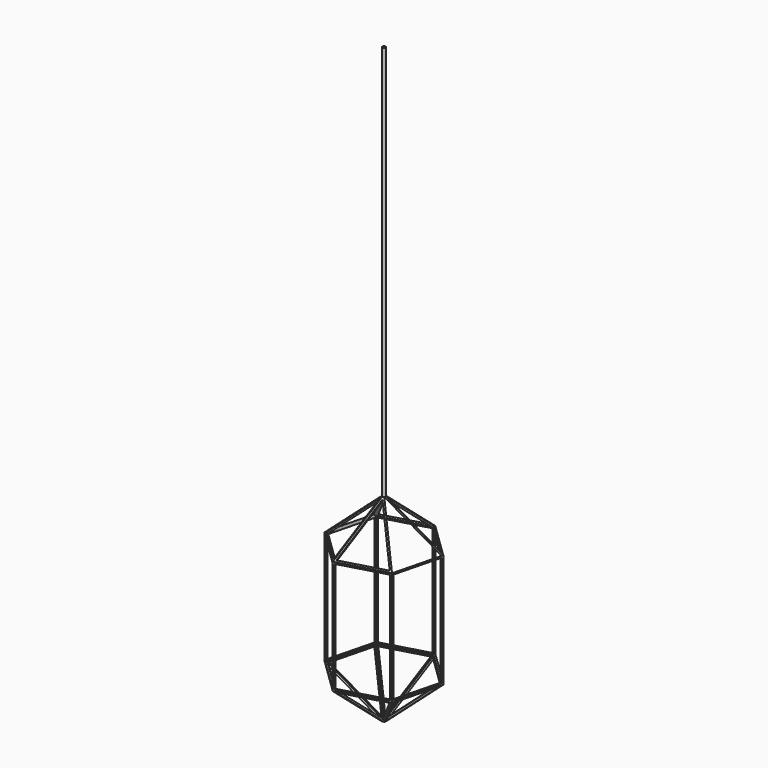
from build123d import *

# Parameters (mm, degrees)
F1_DEPTH  = 300
F2_SIZE   = 63.5
F3_T      = -2.54
F5_DEPTH  = 2.54
F7_DEPTH  = 2.54
F9_DEPTH  = 7.1852048969
F10_DEPTH = 2.541
F12_DEPTH = 2.54
F14_DEPTH = 2.54
F15_W     = 71.12
F15_H     = 167.92
F16_DEPTH = 157.0594794416
F17_W     = 71.12
F17_H     = 167.92
F18_DEPTH = 155.1690173594
F19_W     = 71.12
F19_H     = 167.92
F20_DEPTH = 170.067634702
F22_DEPTH = 2.54
F24_DEPTH = 2.54
F26_DEPTH = 2.54
F28_DEPTH = 2.54
F30_DEPTH = 2.54
F32_DEPTH = 2.54
F33_R     = 2.4911357684
F34_DEPTH = 600


# Not quite as in the source:
# - a feature names something its author has since deleted; it is built from what else it names


with BuildPart() as f1:
    # F0 (on Top) → F1 (new body)
    with BuildSketch(Plane.XY):
        Polygon((73.3134762531, 20.774364002), (18.6656111534, 73.8785148759), (-54.6478650997, 53.104150874), (-73.3134762531, -20.774364002), (-18.6656111534, -73.8785148759), (54.6478650997, -53.104150874), align=None)
    extrude(amount=F1_DEPTH)

    # F2
    f2_edges = [f1.edges().sort_by_distance(p)[0] for p in [
        (45.989544, 47.326439, 300),
        (-17.991127, 63.491333, 300),
        (-63.980671, 16.164893, 300),
        (-45.989544, -47.326439, 300),
        (17.991127, -63.491333, 300),
        (63.980671, -16.164893, 300),
        (45.989544, 47.326439, 0),
        (-17.991127, 63.491333, 0),
        (-63.980671, 16.164893, 0),
        (-45.989544, -47.326439, 0),
        (17.991127, -63.491333, 0),
        (63.980671, -16.164893, 0),
    ]]
    chamfer(f2_edges, length=F2_SIZE)

    # F3
    f3_openings = [f1.faces().sort_by_distance(p)[0] for p in [
        (-42.712352, 10.791394, 258.436633),
    ]]
    offset(amount=F3_T, openings=f3_openings)

    # F4 (on face) → F5 (cut, through all)
    with BuildSketch(Plane(origin=(-105.4037723876, -108.4678135258, 151.2455678842), x_dir=(0.8701504485, -0.287188723, 0.4004507889), z_dir=(-0.4927861574, -0.5071112335, 0.7071067812))):
        Polygon((41.4332766293, 120.899493065), (98.0044622716, 82.0276124879), (117.3270058287, 170.7488222605), align=None)
    extrude(amount=-F5_DEPTH, mode=Mode.SUBTRACT)

    # F6 (on face) → F7 (cut, through all)
    with BuildSketch(Plane(origin=(41.2339958125, -145.5162513053, 151.2455678842), x_dir=(0.9812423716, 0.1336581106, -0.1389205444), z_dir=(0.192778132, -0.6803209476, 0.7071067812))):
        Polygon((-57.8368894269, 113.966214542), (9.4644872932, 127.4512742811), (-40.7019588227, 203.1357603871), align=None)
    extrude(amount=-F7_DEPTH, mode=Mode.SUBTRACT)

    # F8 (on face) → F9 (cut, through all)
    with BuildSketch(Plane(origin=(146.6377682001, -37.0484377795, 151.2455678842), x_dir=(0.7280120913, 0.1631104703, -0.6658778937), z_dir=(0.6855642894, -0.1732097142, 0.7071067812))):
        Polygon((-197.6206426806, 72.1381474707), (-198.5885090871, 69.4293510884), (-126.3576583393, 4.6891971376), (-100.7185084182, 76.4462455114), align=None)
        Polygon((-127.4775404122, 9.1038742336), (-195.0937835337, 69.7079782132), (-104.3824295702, 73.7408450768), align=None, mode=Mode.SUBTRACT)
    extrude(amount=-F9_DEPTH, mode=Mode.SUBTRACT)

    # F8 (on face) + F2_face2 (on face) → F10 (cut, through all)
    with BuildSketch(Plane(origin=(146.6377682001, -37.0484377795, 151.2455678842), x_dir=(0.7280120913, 0.1631104703, -0.6658778937), z_dir=(0.6855642894, -0.1732097142, 0.7071067812))):
        Polygon((-197.6206426806, 72.1381474707), (-198.5885090871, 69.4293510884), (-126.3576583393, 4.6891971376), (-100.7185084182, 76.4462455114), align=None)
        Polygon((-127.4775404122, 9.1038742336), (-195.0937835337, 69.7079782132), (-104.3824295702, 73.7408450768), align=None, mode=Mode.SUBTRACT)
    with BuildSketch(Plane(origin=(42.71235225, -10.7913939511, 258.436632955), x_dir=(0.2449555269, 0.969534316, 0), z_dir=(0.6855642894, -0.1732097142, 0.7071067812))):
        Polygon((0, 55.5822670322), (-34.3195357799, -28.4830838377), (34.3195357799, -28.4830838377), align=None)
    extrude(amount=-F10_DEPTH, mode=Mode.SUBTRACT)

    # F11 (on face) → F12 (cut, through all)
    with BuildSketch(Plane(origin=(105.4037723876, 108.4678135258, 151.2455678842), x_dir=(0.8701504485, -0.287188723, -0.4004507889), z_dir=(0.4927861574, 0.5071112335, 0.7071067812))):
        Polygon((-98.0044622716, -82.0276124879), (-117.3270058287, -170.7488222605), (-41.4332766293, -120.899493065), align=None)
    extrude(amount=-F12_DEPTH, mode=Mode.SUBTRACT)

    # F13 (on face) → F14 (cut, through all)
    with BuildSketch(Plane(origin=(-41.2339958125, 145.5162513053, 151.2455678842), x_dir=(0.9812423716, 0.1336581106, 0.1389205444), z_dir=(-0.192778132, 0.6803209476, 0.7071067812))):
        Polygon((57.8368894269, -113.966214542), (-9.4644872932, -127.4512742811), (40.7019588227, -203.1357603871), align=None)
    extrude(amount=-F14_DEPTH, mode=Mode.SUBTRACT)

    # F15 (on face) → F16 (cut, through all)
    with BuildSketch(Plane(origin=(17.9911269732, -63.4913328749, 0), x_dir=(0.9621191109, 0.2726294488, 0), z_dir=(0.2726294488, -0.9621191109, 0))):
        with Locations((0, 150)):
            Rectangle(F15_W, F15_H)
    extrude(amount=-F16_DEPTH, mode=Mode.SUBTRACT)

    # F17 (on face) → F18 (cut, through all)
    with BuildSketch(Plane(origin=(63.9806706764, -16.164893436, 0), x_dir=(0.2449555269, 0.969534316, 0), z_dir=(0.969534316, -0.2449555269, 0))):
        with Locations((0, 150)):
            Rectangle(F17_W, F17_H)
    extrude(amount=-F18_DEPTH, mode=Mode.SUBTRACT)

    # F19 (on face) → F20 (cut, through all)
    with BuildSketch(Plane(origin=(45.9895437032, 47.3264394389, 0), x_dir=(-0.717163584, 0.6969048671, 0), z_dir=(0.6969048671, 0.717163584, 0))):
        with Locations((0, 150)):
            Rectangle(F19_W, F19_H)
    extrude(amount=-F20_DEPTH, mode=Mode.SUBTRACT)

    # F21 (on face) → F22 (cut, through all)
    with BuildSketch(Plane(origin=(1.2076208066, -0.3051087374, -1.2455678842), x_dir=(0.7280120913, 0.1631104703, 0.6658778937), z_dir=(0.6855642894, -0.1732097142, -0.7071067812))):
        Polygon((95.3809385521, -2.3644010884), (72.2858277101, 62.2725697547), (4.6695845886, 1.6684657751), align=None)
    extrude(amount=-F22_DEPTH, mode=Mode.SUBTRACT)

    # F23 (on face) → F24 (cut, through all)
    with BuildSketch(Plane(origin=(0.8680423208, 0.8932759279, -1.2455678842), x_dir=(0.8701504485, -0.287188723, 0.4004507889), z_dir=(0.4927861574, 0.5071112335, -0.7071067812))):
        Polygon((22.13077439, -92.8080958564), (78.7019600324, -53.9362152793), (2.808230833, -4.0868860838), align=None)
    extrude(amount=-F24_DEPTH, mode=Mode.SUBTRACT)

    # F25 (on face) → F26 (cut, through all)
    with BuildSketch(Plane(origin=(-0.3395784858, 1.1983846653, -1.2455678842), x_dir=(0.9812423716, 0.1336581106, -0.1389205444), z_dir=(-0.192778132, 0.6803209476, -0.7071067812))):
        Polygon((16.1607261154, -94.0316157631), (-0.9742044888, -4.862069918), (-51.1406506047, -80.546556024), align=None)
    extrude(amount=-F26_DEPTH, mode=Mode.SUBTRACT)

    # F27 (on face) → F28 (cut, through all)
    with BuildSketch(Plane(origin=(-1.2076208066, 0.3051087374, -1.2455678842), x_dir=(0.7280120913, 0.1631104703, -0.6658778937), z_dir=(-0.6855642894, 0.1732097142, -0.7071067812))):
        Polygon((-72.2858277101, -62.2725697547), (-4.6695845886, -1.6684657751), (-95.3809385521, 2.3644010884), align=None)
    extrude(amount=-F28_DEPTH, mode=Mode.SUBTRACT)

    # F29 (on face) → F30 (cut, through all)
    with BuildSketch(Plane(origin=(-0.8680423208, -0.8932759279, -1.2455678842), x_dir=(0.8701504485, -0.287188723, -0.4004507889), z_dir=(-0.4927861574, -0.5071112335, -0.7071067812))):
        Polygon((-78.7019600324, 53.9362152793), (-2.808230833, 4.0868860838), (-22.13077439, 92.8080958564), align=None)
    extrude(amount=-F30_DEPTH, mode=Mode.SUBTRACT)

    # F31 (on face) → F32 (cut, through all)
    with BuildSketch(Plane(origin=(0.3395784858, -1.1983846653, -1.2455678842), x_dir=(0.9812423716, 0.1336581106, 0.1389205444), z_dir=(0.192778132, -0.6803209476, -0.7071067812))):
        Polygon((-16.1607261154, 94.0316157631), (0.9742044888, 4.862069918), (51.1406506047, 80.546556024), align=None)
    extrude(amount=-F32_DEPTH, mode=Mode.SUBTRACT)

    # F33 (on face) → F34 (join)
    with BuildSketch(Plane.XY.offset(300)):
        Circle(F33_R)
    extrude(amount=F34_DEPTH)


solid = f1.part
